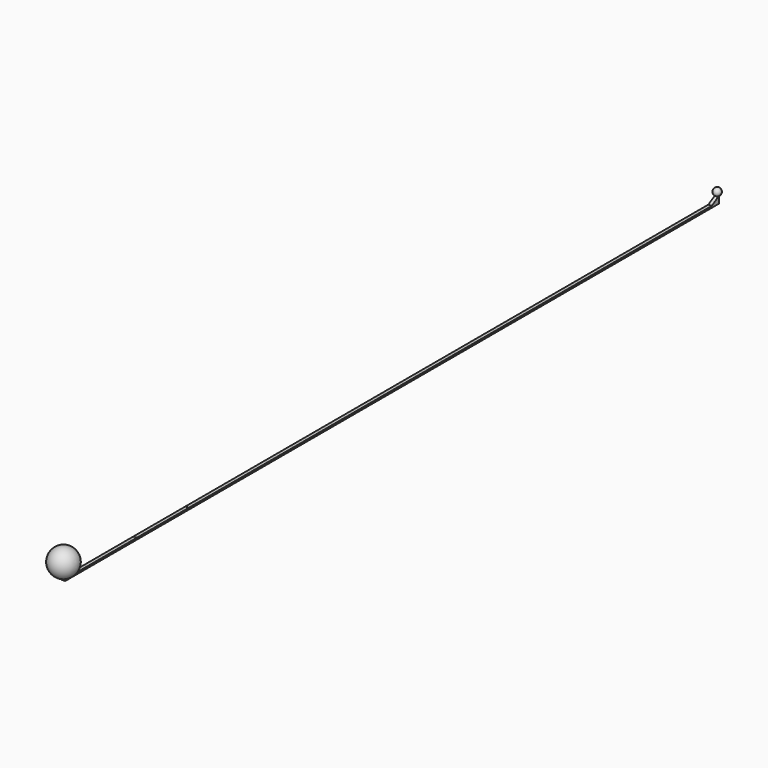
from build123d import *

# Parameters (mm, degrees)
F2_W          = 6045.2
F2_H          = 12.7
F3_DEPTH      = 12.7
F7_DEPTH      = 12.7
F7_DEPTH_BACK = 12.7
F8_DEPTH      = 12.7
F9_W          = 25.4
F9_H          = 2.54
F10_DEPTH     = 2.54
F11_TEXT_SIZE = 3.5277777778
F12_DEPTH     = 2.54
F13_W         = 2.54
F13_H         = 2.54
F14_DEPTH     = 113.25325
F15_TEXT_SIZE = 3.5277777778
F16_DEPTH     = 2.54
F17_W         = 2.54
F17_H         = 2.54
F18_DEPTH     = 25.4
F19_TEXT_SIZE = 3.5277777778
F20_DEPTH     = 2.54


# Not quite as in the source:
# - Text() gives the source's letters only with a copy of the font that has no kerning and outlines rounded to 1/6400 em; it was checked with that copy


with BuildPart() as f1:
    # F0 (on Front) → F1 (revolve)
    with BuildSketch(Plane.XZ):
        with BuildLine():
            Line((0, 0), (0, -100.55225))
            ThreePointArc((0, -100.55225), (100.55225, 0), (0, 100.55225))
            Line((0, 100.55225), (0, 0))
        make_face()
    revolve(axis=Axis((0, 0, 60.7964061201), (0, 0, 1)))



with BuildPart() as f3:
    # F2 (on Right) → F3 (new body)
    with BuildSketch(Plane.YZ):
        with Locations((3022.6, -114.3)):
            Rectangle(F2_W, F2_H)
    extrude(amount=F3_DEPTH)


with BuildPart() as f5:
    # F4 (on face) → F5 (revolve)
    with BuildSketch(Plane(origin=(0, 0, 0), x_dir=(0, -1, 0), z_dir=(-1, 0, 0))):
        with BuildLine():
            Line((-6045.0204900531, -19.0501585819), (-6045.1173805469, -73.8886729873))
            ThreePointArc((-6045.1173805469, -73.8886729873), (-6017.6496780973, -46.5178610315), (-6045.0204900531, -19.0501585819))
        make_face()
    revolve(axis=Axis((0, 6045.1102450266, -69.850079291), (0, -0.0017668302, 0.9999984392)))


with BuildPart() as f1_1:
    add(f1.part)

    add(f3.part)  # F7 merges F3

    add(f5.part)  # F7 merges F5
    # F6 (on face) → F7 (join, two sides)
    with BuildSketch(Plane(origin=(0, 0, 0), x_dir=(0, -1, 0), z_dir=(-1, 0, 0))) as f7_sk:
        Polygon((-6045.2, -69.85), (-6045.2, -120.65), (-5957.2118189755, -120.65), align=None)
        Polygon((-87.9881810245, -120.65), (0, -120.65), (0, -69.85), align=None)
    extrude(amount=F7_DEPTH)
    extrude(f7_sk.sketch, amount=-F7_DEPTH_BACK)

    # F8 (add): a face of the model
    f8_faces = [f1_1.faces().sort_by_distance(p)[0] for p in [
        (0, 3022.6, -114.2920966443),
    ]]
    extrude(f8_faces, amount=F8_DEPTH)

    # F9 (on face) → F10 (cut)
    with BuildSketch(Plane.XY.offset(-107.95)):
        with Locations((0, 102.87)):
            Rectangle(F9_W, F9_H)
    extrude(amount=-F10_DEPTH, mode=Mode.SUBTRACT)

    # F11 (on face) → F12 (cut)
    with BuildSketch(Plane.YZ.offset(12.7)):
        with Locations((90.3978458378, -113.665)):
            Text('Low Earth Orbit', F11_TEXT_SIZE, font='Open Sans', text_align=(TextAlign.LEFT, TextAlign.BOTTOM))
        with Locations((81.2311357684, -118.4627777778)):
            Text('(International Space Station)', F11_TEXT_SIZE, font='Open Sans', text_align=(TextAlign.LEFT, TextAlign.BOTTOM))
    extrude(amount=-F12_DEPTH, mode=Mode.SUBTRACT)

    # F13 (on face) → F14 (cut, through all)
    with BuildSketch(Plane.YZ.offset(12.7)):
        with Locations((661.67, -109.22)):
            Rectangle(F13_W, F13_H)
    extrude(amount=-F14_DEPTH, mode=Mode.SUBTRACT)

    # F15 (on face) → F16 (cut)
    with BuildSketch(Plane.YZ.offset(12.7)):
        with Locations((642.1233550347, -113.665)):
            Text('Geosynchronous Orbit', F15_TEXT_SIZE, font='Open Sans', text_align=(TextAlign.LEFT, TextAlign.BOTTOM))
        with Locations((637.54, -118.4627777778)):
            Text('(GPS and Television Satellites)', F15_TEXT_SIZE, font='Open Sans', text_align=(TextAlign.LEFT, TextAlign.BOTTOM))
    extrude(amount=-F16_DEPTH, mode=Mode.SUBTRACT)

    # F17 (on face) → F18 (cut)
    with BuildSketch(Plane.YZ.offset(12.7)):
        with Locations((1144.27, -109.22)):
            Rectangle(F17_W, F17_H)
    extrude(amount=-F18_DEPTH, mode=Mode.SUBTRACT)

    # F19 (on face) → F20 (cut)
    with BuildSketch(Plane.YZ.offset(12.7)):
        with Locations((1132.8802387153, -113.665)):
            Text('Van Allen Belt', F19_TEXT_SIZE, font='Open Sans', text_align=(TextAlign.LEFT, TextAlign.BOTTOM))
    extrude(amount=-F20_DEPTH, mode=Mode.SUBTRACT)


solid = f1_1.part
